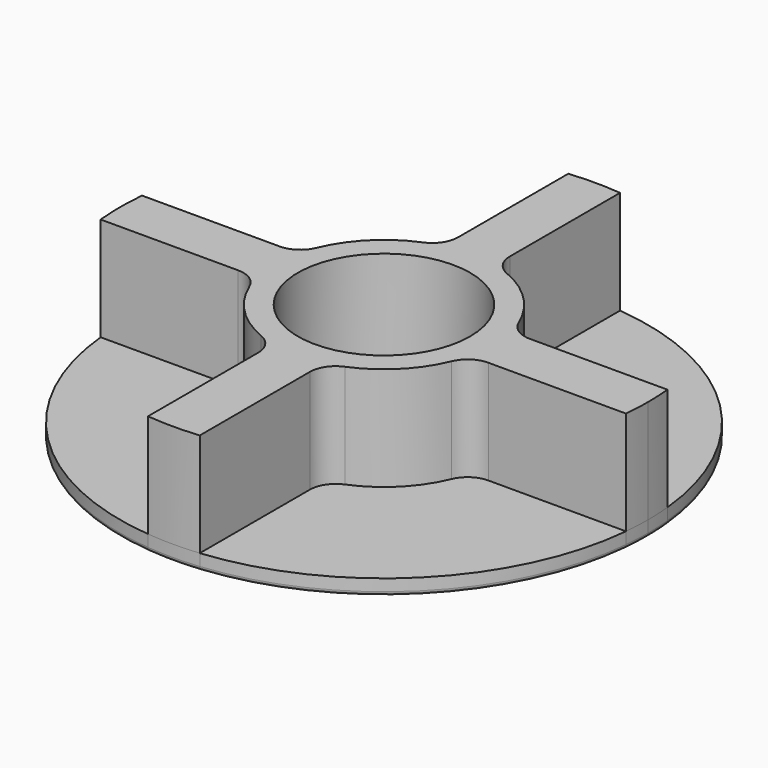
from build123d import *

# Parameters (mm, degrees)
F0_R     = 6.65
F0_R_2   = 2.55
F1_DEPTH = 1.2
F2_DEPTH = 8
F3_R     = 0.3


# Not quite as in the source:
# - a feature names something its author has since deleted; it is built from what else it names


with BuildPart() as f1:
    # F0 (on Top) → F1 (new body)
    with BuildSketch(Plane.XY):
        with BuildLine():
            Line((9.6529388756, 1.998378199), (20.2717385681, 1.998378199))
            ThreePointArc((20.2717385681, 1.998378199), (14.4037651328, 14.4037651328), (1.998378199, 20.2717385681))
            Line((1.998378199, 20.2717385681), (1.998378199, 9.6529388756))
            ThreePointArc((1.998378199, 9.6529388756), (2.3354389744, 8.5417984096), (3.2330113343, 7.8051798106))
            ThreePointArc((3.2330113343, 7.8051798106), (5.9738260003, 5.9738260003), (7.8051798106, 3.2330113343))
            ThreePointArc((7.8051798106, 3.2330113343), (8.5417984096, 2.3354389744), (9.6529388756, 1.998378199))
        make_face()
        with BuildLine():
            Line((-1.998378199, 9.6529388756), (-1.998378199, 20.2717385681))
            ThreePointArc((-1.998378199, 20.2717385681), (-14.4037651328, 14.4037651328), (-20.2717385681, 1.998378199))
            Line((-20.2717385681, 1.998378199), (-9.6529388756, 1.998378199))
            ThreePointArc((-9.6529388756, 1.998378199), (-8.5417984096, 2.3354389744), (-7.8051798106, 3.2330113343))
            ThreePointArc((-7.8051798106, 3.2330113343), (-5.9738260003, 5.9738260003), (-3.2330113343, 7.8051798106))
            ThreePointArc((-3.2330113343, 7.8051798106), (-2.3354389744, 8.5417984096), (-1.998378199, 9.6529388756))
        make_face()
        with BuildLine():
            ThreePointArc((-20.2717385681, -1.998378199), (-14.4037651328, -14.4037651328), (-1.998378199, -20.2717385681))
            Line((-1.998378199, -20.2717385681), (-1.998378199, -9.6529388756))
            ThreePointArc((-1.998378199, -9.6529388756), (-2.3354389744, -8.5417984096), (-3.2330113343, -7.8051798106))
            ThreePointArc((-3.2330113343, -7.8051798106), (-5.9738260003, -5.9738260003), (-7.8051798106, -3.2330113343))
            ThreePointArc((-7.8051798106, -3.2330113343), (-8.5417984096, -2.3354389744), (-9.6529388756, -1.998378199))
            Line((-9.6529388756, -1.998378199), (-20.2717385681, -1.998378199))
        make_face()
        with BuildLine():
            ThreePointArc((1.998378199, -20.2717385681), (14.4037651328, -14.4037651328), (20.2717385681, -1.998378199))
            Line((20.2717385681, -1.998378199), (9.6529388756, -1.998378199))
            ThreePointArc((9.6529388756, -1.998378199), (8.5417984096, -2.3354389744), (7.8051798106, -3.2330113343))
            ThreePointArc((7.8051798106, -3.2330113343), (5.9738260003, -5.9738260003), (3.2330113343, -7.8051798106))
            ThreePointArc((3.2330113343, -7.8051798106), (2.3354389744, -8.5417984096), (1.998378199, -9.6529388756))
            Line((1.998378199, -9.6529388756), (1.998378199, -20.2717385681))
        make_face()
        with BuildLine():
            ThreePointArc((20.2717385681, -1.998378199), (20.3454198117, -1.0003962634), (20.37, 0))
            ThreePointArc((20.37, 0), (20.3454198117, 1.0003962634), (20.2717385681, 1.998378199))
            Line((20.2717385681, 1.998378199), (9.6529388756, 1.998378199))
            ThreePointArc((9.6529388756, 1.998378199), (8.5417984096, 2.3354389744), (7.8051798106, 3.2330113343))
            ThreePointArc((7.8051798106, 3.2330113343), (5.9738260003, 5.9738260003), (3.2330113343, 7.8051798106))
            ThreePointArc((3.2330113343, 7.8051798106), (2.3354389744, 8.5417984096), (1.998378199, 9.6529388756))
            Line((1.998378199, 9.6529388756), (1.998378199, 20.2717385681))
            ThreePointArc((1.998378199, 20.2717385681), (0, 20.37), (-1.998378199, 20.2717385681))
            Line((-1.998378199, 20.2717385681), (-1.998378199, 9.6529388756))
            ThreePointArc((-1.998378199, 9.6529388756), (-2.3354389744, 8.5417984096), (-3.2330113343, 7.8051798106))
            ThreePointArc((-3.2330113343, 7.8051798106), (-5.9738260003, 5.9738260003), (-7.8051798106, 3.2330113343))
            ThreePointArc((-7.8051798106, 3.2330113343), (-8.5417984096, 2.3354389744), (-9.6529388756, 1.998378199))
            Line((-9.6529388756, 1.998378199), (-20.2717385681, 1.998378199))
            ThreePointArc((-20.2717385681, 1.998378199), (-20.37, 0), (-20.2717385681, -1.998378199))
            Line((-20.2717385681, -1.998378199), (-9.6529388756, -1.998378199))
            ThreePointArc((-9.6529388756, -1.998378199), (-8.5417984096, -2.3354389744), (-7.8051798106, -3.2330113343))
            ThreePointArc((-7.8051798106, -3.2330113343), (-5.9738260003, -5.9738260003), (-3.2330113343, -7.8051798106))
            ThreePointArc((-3.2330113343, -7.8051798106), (-2.3354389744, -8.5417984096), (-1.998378199, -9.6529388756))
            Line((-1.998378199, -9.6529388756), (-1.998378199, -20.2717385681))
            ThreePointArc((-1.998378199, -20.2717385681), (0, -20.37), (1.998378199, -20.2717385681))
            Line((1.998378199, -20.2717385681), (1.998378199, -9.6529388756))
            ThreePointArc((1.998378199, -9.6529388756), (2.3354389744, -8.5417984096), (3.2330113343, -7.8051798106))
            ThreePointArc((3.2330113343, -7.8051798106), (5.9738260003, -5.9738260003), (7.8051798106, -3.2330113343))
            ThreePointArc((7.8051798106, -3.2330113343), (8.5417984096, -2.3354389744), (9.6529388756, -1.998378199))
            Line((9.6529388756, -1.998378199), (20.2717385681, -1.998378199))
        make_face()
        Circle(F0_R, mode=Mode.SUBTRACT)
        Circle(F0_R)
        Circle(F0_R_2, mode=Mode.SUBTRACT)
    extrude(amount=-F1_DEPTH)

    # F0 (on Top) → F2 (join)
    with BuildSketch(Plane.XY):
        with BuildLine():
            ThreePointArc((20.2717385681, -1.998378199), (20.3454198117, -1.0003962634), (20.37, 0))
            ThreePointArc((20.37, 0), (20.3454198117, 1.0003962634), (20.2717385681, 1.998378199))
            Line((20.2717385681, 1.998378199), (9.6529388756, 1.998378199))
            ThreePointArc((9.6529388756, 1.998378199), (8.5417984096, 2.3354389744), (7.8051798106, 3.2330113343))
            ThreePointArc((7.8051798106, 3.2330113343), (5.9738260003, 5.9738260003), (3.2330113343, 7.8051798106))
            ThreePointArc((3.2330113343, 7.8051798106), (2.3354389744, 8.5417984096), (1.998378199, 9.6529388756))
            Line((1.998378199, 9.6529388756), (1.998378199, 20.2717385681))
            ThreePointArc((1.998378199, 20.2717385681), (0, 20.37), (-1.998378199, 20.2717385681))
            Line((-1.998378199, 20.2717385681), (-1.998378199, 9.6529388756))
            ThreePointArc((-1.998378199, 9.6529388756), (-2.3354389744, 8.5417984096), (-3.2330113343, 7.8051798106))
            ThreePointArc((-3.2330113343, 7.8051798106), (-5.9738260003, 5.9738260003), (-7.8051798106, 3.2330113343))
            ThreePointArc((-7.8051798106, 3.2330113343), (-8.5417984096, 2.3354389744), (-9.6529388756, 1.998378199))
            Line((-9.6529388756, 1.998378199), (-20.2717385681, 1.998378199))
            ThreePointArc((-20.2717385681, 1.998378199), (-20.37, 0), (-20.2717385681, -1.998378199))
            Line((-20.2717385681, -1.998378199), (-9.6529388756, -1.998378199))
            ThreePointArc((-9.6529388756, -1.998378199), (-8.5417984096, -2.3354389744), (-7.8051798106, -3.2330113343))
            ThreePointArc((-7.8051798106, -3.2330113343), (-5.9738260003, -5.9738260003), (-3.2330113343, -7.8051798106))
            ThreePointArc((-3.2330113343, -7.8051798106), (-2.3354389744, -8.5417984096), (-1.998378199, -9.6529388756))
            Line((-1.998378199, -9.6529388756), (-1.998378199, -20.2717385681))
            ThreePointArc((-1.998378199, -20.2717385681), (0, -20.37), (1.998378199, -20.2717385681))
            Line((1.998378199, -20.2717385681), (1.998378199, -9.6529388756))
            ThreePointArc((1.998378199, -9.6529388756), (2.3354389744, -8.5417984096), (3.2330113343, -7.8051798106))
            ThreePointArc((3.2330113343, -7.8051798106), (5.9738260003, -5.9738260003), (7.8051798106, -3.2330113343))
            ThreePointArc((7.8051798106, -3.2330113343), (8.5417984096, -2.3354389744), (9.6529388756, -1.998378199))
            Line((9.6529388756, -1.998378199), (20.2717385681, -1.998378199))
        make_face()
        Circle(F0_R, mode=Mode.SUBTRACT)
    extrude(amount=F2_DEPTH)

    # F3
    f3_edges = [f1.edges().sort_by_distance(p)[0] for p in [
        (-1.998378, -20.271739, -1.2),
    ]]
    fillet(f3_edges, radius=F3_R)


solid = f1.part
